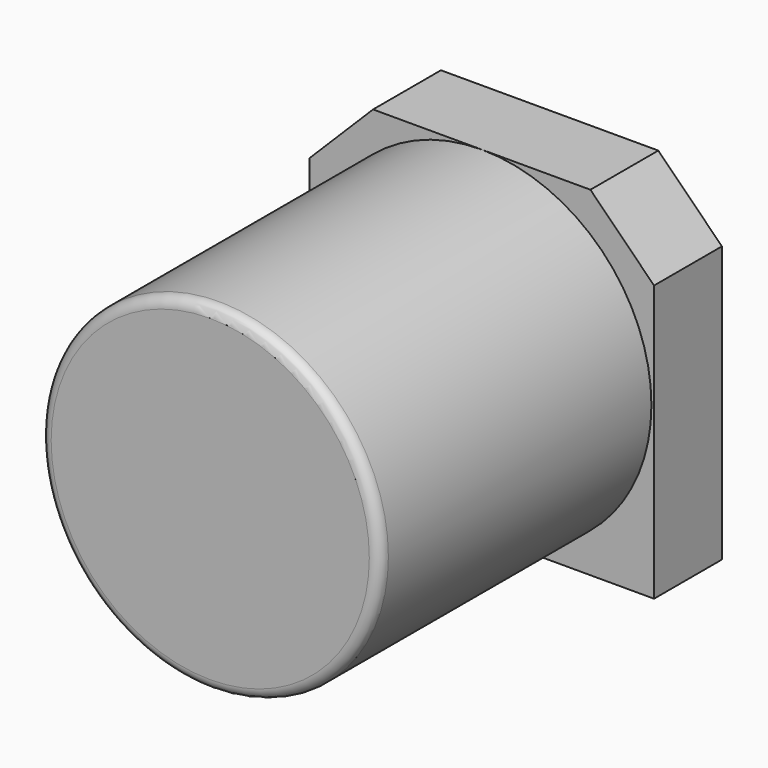
from build123d import *

# Parameters (mm, degrees)
F0_R     = 3.175
F1_DEPTH = 6.35
F3_DEPTH = 1.5875
F4_R     = 0.1984375


with BuildPart() as f1:
    # F0 (on Front) → F1 (new body)
    with BuildSketch(Plane.XZ):
        Circle(F0_R)
    extrude(amount=F1_DEPTH)

    # F2 (on face) → F3 (join)
    with BuildSketch(Plane(origin=(0, 0, 0), x_dir=(-1, 0, 0), z_dir=(0, 1, 0))):
        with BuildLine():
            Line((0, 3.175), (-2.033528515, 3.175))
            Line((-2.033528515, 3.175), (-3.224153515, 1.984375))
            Line((-3.224153515, 1.984375), (-3.224153515, -3.175))
            Line((-3.224153515, -3.175), (0, -3.175))
            ThreePointArc((0, -3.175), (-3.175, 0), (0, 3.175))
        make_face()
        with BuildLine():
            Line((2.033528515, 3.175), (0, 3.175))
            ThreePointArc((0, 3.175), (2.2450640303, 2.2450640303), (3.175, 0))
            ThreePointArc((3.175, 0), (2.2450640303, -2.2450640303), (0, -3.175))
            Line((0, -3.175), (3.224153515, -3.175))
            Line((3.224153515, -3.175), (3.224153515, 1.984375))
            Line((3.224153515, 1.984375), (2.033528515, 3.175))
        make_face()
        with BuildLine():
            ThreePointArc((3.175, 0), (2.2450640303, 2.2450640303), (0, 3.175))
            ThreePointArc((0, 3.175), (-3.175, 0), (0, -3.175))
            ThreePointArc((0, -3.175), (2.2450640303, -2.2450640303), (3.175, 0))
        make_face()
    extrude(amount=F3_DEPTH)

    # F4
    f4_edges = [f1.edges().sort_by_distance(p)[0] for p in [
        (-3.175, -6.35, 0),
    ]]
    fillet(f4_edges, radius=F4_R)


solid = f1.part
